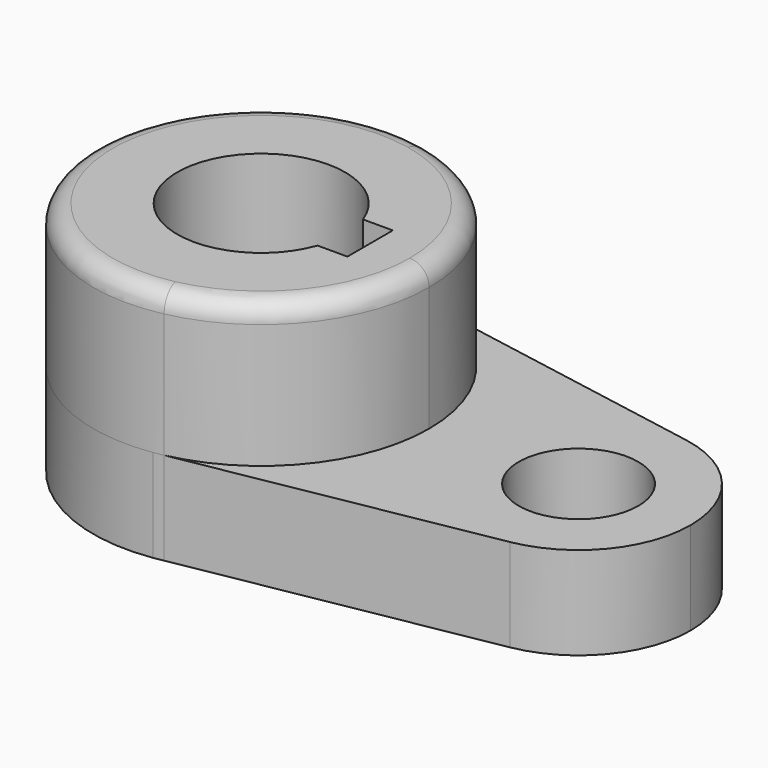
from build123d import *
from build123d import SkipClean  # not in build123d's __all__

# Parameters (mm, degrees)
F0_R     = 10.16
F1_DEPTH = 15.7734
F3_DEPTH = 24.4602
F4_R     = 3.302


with BuildPart() as f1:
    # F0 (on Top) → F1 (new body)
    with BuildSketch(Plane.XY):
        with BuildLine():
            Line((5.865458004, 27.9665340613), (4.2022058824, 28.2643254072))
            ThreePointArc((4.2022058824, 28.2643254072), (-28.575, 0), (4.2022058824, -28.2643254072))
            Line((4.2022058824, -28.2643254072), (5.865458004, -27.9665340613))
            ThreePointArc((5.865458004, -27.9665340613), (22.182606784, -18.0128448966), (28.575, 0))
            ThreePointArc((28.575, 0), (22.182606784, 18.0128448966), (5.865458004, 27.9665340613))
        make_face()
        with BuildLine():
            ThreePointArc((13.4477648793, -4.826), (-14.2875, 0), (13.4477648793, 4.826))
            Line((13.4477648793, 4.826), (18.5293, 4.826))
            Line((18.5293, 4.826), (18.5293, -4.826))
            Line((18.5293, -4.826), (13.4477648793, -4.826))
        make_face(mode=Mode.SUBTRACT)
        with BuildLine():
            ThreePointArc((5.865458004, 27.9665340613), (5.0360335537, 28.1277263753), (4.2022058824, 28.2643254072))
            Line((4.2022058824, 28.2643254072), (5.865458004, 27.9665340613))
        make_face()
        with BuildLine():
            Line((5.865458004, -27.9665340613), (4.2022058824, -28.2643254072))
            ThreePointArc((4.2022058824, -28.2643254072), (5.0360335537, -28.1277263753), (5.865458004, -27.9665340613))
        make_face()
        with BuildLine():
            Line((57.3323557024, 18.7518175836), (5.865458004, 27.9665340613))
            ThreePointArc((5.865458004, 27.9665340613), (22.182606784, 18.0128448966), (28.575, 0))
            ThreePointArc((28.575, 0), (22.182606784, -18.0128448966), (5.865458004, -27.9665340613))
            Line((5.865458004, -27.9665340613), (57.3323557024, -18.7518175836))
            ThreePointArc((57.3323557024, -18.7518175836), (34.925, 0), (57.3323557024, 18.7518175836))
        make_face()
        with BuildLine():
            ThreePointArc((73.025, 0), (68.5842458076, 12.2258920711), (57.3323557024, 18.7518175836))
            ThreePointArc((57.3323557024, 18.7518175836), (34.925, 0), (57.3323557024, -18.7518175836))
            ThreePointArc((57.3323557024, -18.7518175836), (68.5842458076, -12.2258920711), (73.025, 0))
        make_face()
        with Locations((53.975, 0)):
            Circle(F0_R, mode=Mode.SUBTRACT)
    extrude(amount=-F1_DEPTH)

    # F2 (on face) → F3 (join)
    with BuildSketch(Plane.XY):
        with BuildLine():
            ThreePointArc((28.575, 0), (22.182606784, 18.0128448966), (5.865458004, 27.9665340613))
            ThreePointArc((5.865458004, 27.9665340613), (-28.575, 0), (5.865458004, -27.9665340613))
            ThreePointArc((5.865458004, -27.9665340613), (22.182606784, -18.0128448966), (28.575, 0))
        make_face()
        with BuildLine():
            ThreePointArc((13.4477648793, -4.826), (-14.2875, 0), (13.4477648793, 4.826))
            Line((13.4477648793, 4.826), (18.5293, 4.826))
            Line((18.5293, 4.826), (18.5293, -4.826))
            Line((18.5293, -4.826), (13.4477648793, -4.826))
        make_face(mode=Mode.SUBTRACT)
    with SkipClean():  # cleaning this boolean's faces spoils the solid; the shape is the same uncleaned
        extrude(amount=F3_DEPTH)

    # F4
    f4_edges = [f1.edges().sort_by_distance(p)[0] for p in [
        (-5.865458, 27.966534, 24.4602),
    ]]
    fillet(f4_edges, radius=F4_R)


solid = f1.part
